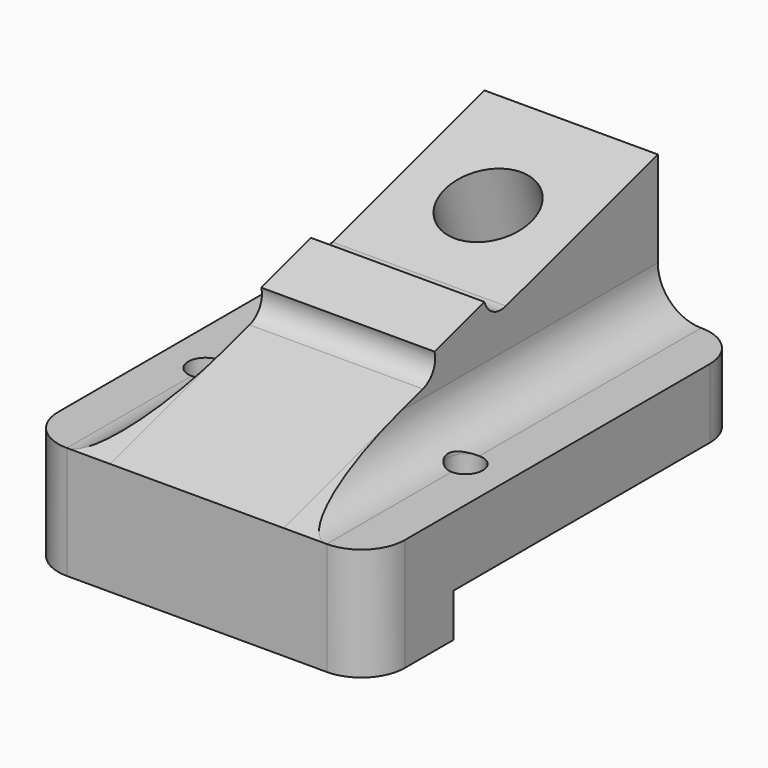
from build123d import *

# Parameters (mm, degrees)
F1_DEPTH     = 20
F2_DEPTH     = 40
F3_T4_DEPTH  = 108
F3_T9_DEPTH  = 108
F3_T11_DEPTH = 76
F3_T13_DEPTH = 66
F4_R         = 10
F5_DEPTH     = 25
F6_R         = 4
F7_DEPTH     = 16
F8_DEPTH     = 25


# Not quite as in the source:
# - a fillet or chamfer that OpenCascade refuses, or shapes differently, is made with other operations: its cross-section is extruded or revolved along the edge and cut away or added


with BuildPart() as f1:
    # F0 (on Right) → F1 (new body, symmetric)
    with BuildSketch(Plane.YZ):
        with BuildLine():
            Line((40.2060094365, 37.9128916849), (0, 26))
            Line((0, 26), (108, 26))
            Line((108, 26), (108, 58))
            Line((108, 58), (64.1759622542, 45.0150999272))
            ThreePointArc((64.1759622542, 45.0150999272), (60.3700612912, 45.4148233324), (57.9615300422, 48.3886488422))
            Line((57.9615300422, 48.3886488422), (43.5795583515, 44.1273238969))
            ThreePointArc((43.5795583515, 44.1273238969), (43.1798349463, 40.3214229339), (40.2060094365, 37.9128916849))
        make_face()
    extrude(amount=F1_DEPTH, both=True)

    # F0 (on Right) → F2 (join, symmetric)
    with BuildSketch(Plane.YZ):
        Polygon((0, 26), (0, 0), (24, 0), (24, 10), (108, 10), (108, 26), align=None)
    extrude(amount=F2_DEPTH, both=True)

    # F3: fillet of radius 10 on 6 edges, made by hand


with BuildPart() as f3_tool2:
    # F3_s3 → F3_t4 (new body)
    with BuildSketch(Plane.XZ):
        with BuildLine():
            ThreePointArc((30, 26), (22.9289321881, 28.9289321881), (20, 36))
            Line((20, 36), (20, 26))
            Line((20, 26), (30, 26))
        make_face()
    extrude(amount=-F3_T4_DEPTH)

    split(bisect_by=Plane(origin=(0, -7.0819672131, 23.9016393443), x_dir=(1, 0, 0), z_dir=(0, 0.2840883297, -0.9587981127)), keep=Keep.TOP)


with BuildPart() as f1_1:
    add(f1.part)

    # F3_t1: union F3_tool2
    add(f3_tool2.part)


with BuildPart() as f3_tool7:
    # F3_s8 → F3_t9 (new body)
    with BuildSketch(Plane.XZ):
        with BuildLine():
            ThreePointArc((-30, 26), (-22.9289321881, 28.9289321881), (-20, 36))
            Line((-20, 36), (-20, 26))
            Line((-20, 26), (-30, 26))
        make_face()
    extrude(amount=-F3_T9_DEPTH)

    split(bisect_by=Plane(origin=(0, -7.0819672131, 23.9016393443), x_dir=(1, 0, 0), z_dir=(0, 0.2840883297, -0.9587981127)), keep=Keep.TOP)


with BuildPart() as f1_2:
    add(f1_1.part)

    # F3_t6: union F3_tool7
    add(f3_tool7.part)

    # F3_s12 → F3_t11 (cut)
    with BuildSketch(Plane.XY.offset(-25)):
        with BuildLine():
            ThreePointArc((30, 0), (37.0710678119, 2.9289321881), (40, 10))
            Line((40, 10), (40, 0))
            Line((40, 0), (30, 0))
        make_face()
        with BuildLine():
            ThreePointArc((-30, 0), (-37.0710678119, 2.9289321881), (-40, 10))
            Line((-40, 10), (-40, 0))
            Line((-40, 0), (-30, 0))
        make_face()
    extrude(amount=F3_T11_DEPTH, mode=Mode.SUBTRACT)

    # F3_s14 → F3_t13 (cut)
    with BuildSketch(Plane.XY.offset(-15)):
        with BuildLine():
            ThreePointArc((30, 108), (37.0710678119, 105.0710678119), (40, 98))
            Line((40, 98), (40, 108))
            Line((40, 108), (30, 108))
        make_face()
        with BuildLine():
            ThreePointArc((-30, 108), (-37.0710678119, 105.0710678119), (-40, 98))
            Line((-40, 98), (-40, 108))
            Line((-40, 108), (-30, 108))
        make_face()
    extrude(amount=F3_T13_DEPTH, mode=Mode.SUBTRACT)

    # F4 (on face) → F5 (cut)
    with BuildSketch(Plane(origin=(0, -7.0819672131, 23.9016393443), x_dir=(1, 0, 0), z_dir=(0, -0.2840883297, 0.9587981127))):
        with Locations((0, 95.0273192946)):
            Circle(F4_R)
    extrude(amount=-F5_DEPTH, mode=Mode.SUBTRACT)

    # F6 (on face) → F7 (cut, through all)
    with BuildSketch(Plane.XY.offset(26)):
        with Locations((30, 40)):
            Circle(F6_R)
        with Locations((-30, 40)):
            Circle(F6_R)
    extrude(amount=-F7_DEPTH, mode=Mode.SUBTRACT)

    # F6 (on face) → F8 (cut)
    with BuildSketch(Plane.XY.offset(26)):
        with Locations((30, 40)):
            Circle(F6_R)
        with Locations((-30, 40)):
            Circle(F6_R)
    extrude(amount=F8_DEPTH, mode=Mode.SUBTRACT)


solid = f1_2.part
